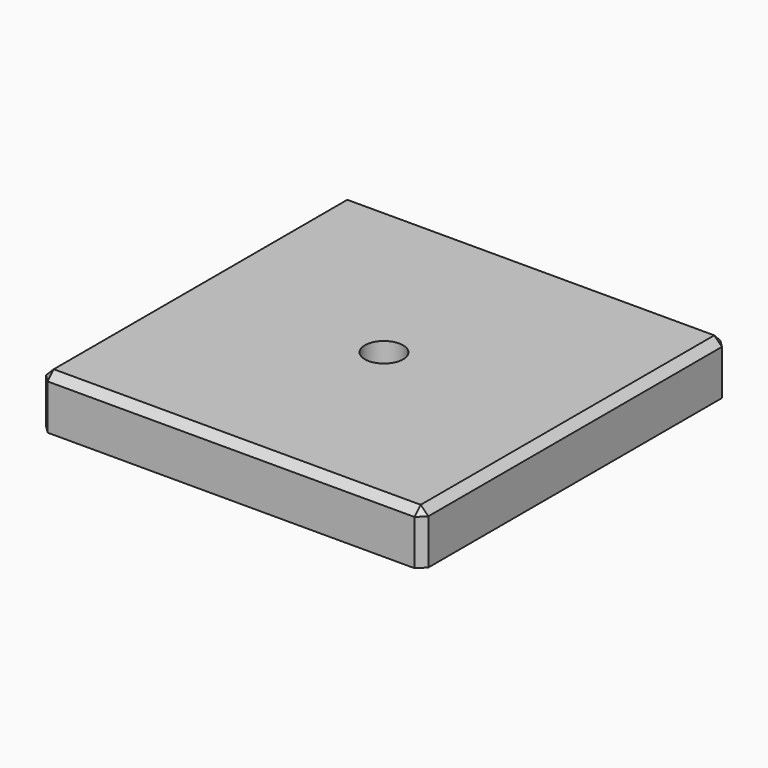
from build123d import *

# Parameters (mm, degrees)
F0_W     = 500
F0_H     = 500
F0_R     = 25
F1_DEPTH = 19
F2_W     = 500
F2_H     = 500
F2_W_2   = 462
F2_H_2   = 462
F2_W_3   = 120
F2_H_3   = 120
F2_R     = 25
F3_DEPTH = 50
F4_SIZE  = 10


with BuildPart() as f1:
    # F0 (on Top) → F1 (new body)
    with BuildSketch(Plane.XY):
        Rectangle(F0_W, F0_H)
        Circle(F0_R, mode=Mode.SUBTRACT)
    extrude(amount=F1_DEPTH)

    # F2 (on face) → F3 (join)
    with BuildSketch(Plane(origin=(0, 0, 0), x_dir=(1, 0, 0), z_dir=(0, 0, -1))):
        Rectangle(F2_W, F2_H)
        Rectangle(F2_W_2, F2_H_2, mode=Mode.SUBTRACT)
        Rectangle(F2_W_3, F2_H_3)
        Circle(F2_R, mode=Mode.SUBTRACT)
    extrude(amount=F3_DEPTH)

    # F4
    f4_edges = [f1.edges().sort_by_distance(p)[0] for p in [
        (0, 250, 19),
        (250, 0, 19),
        (0, -250, 19),
        (-250, 0, 19),
        (-250, 250, -15.5),
        (-250, -250, -15.5),
        (250, 250, -15.5),
        (250, -250, -15.5),
    ]]
    chamfer(f4_edges, length=F4_SIZE)


solid = f1.part
